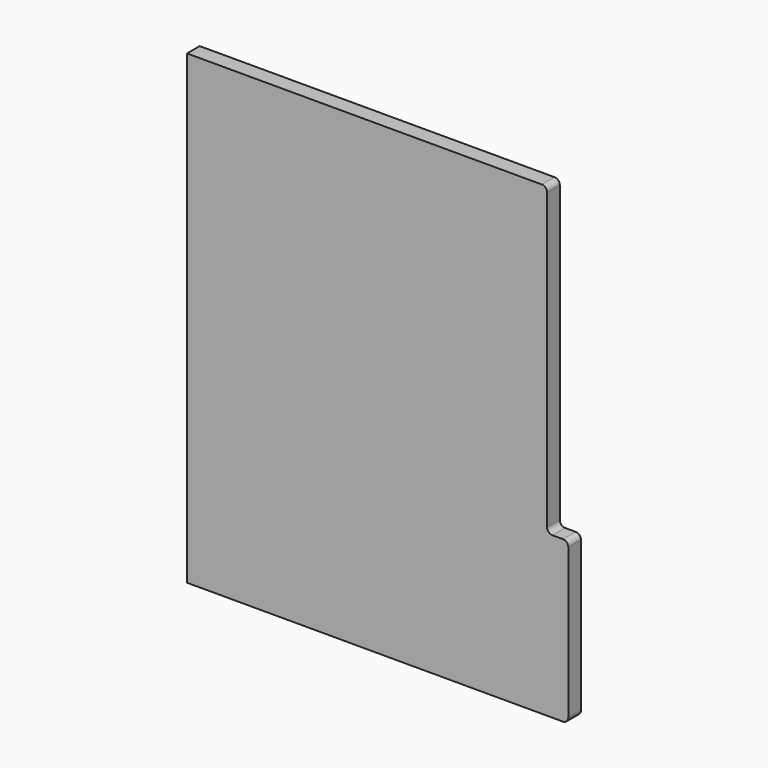
from build123d import *

# Parameters (mm, degrees)
F0_W     = 215.9
F0_H     = 279.4
F1_DEPTH = 9.525
F2_W     = 12.7
F2_H     = 96.3083333333
F3_DEPTH = 9.525
F4_R     = 3.175


with BuildPart() as f1:
    # F0 (on Front) → F1 (new body)
    with BuildSketch(Plane.XZ):
        Rectangle(F0_W, F0_H)
    extrude(amount=F1_DEPTH)

    # F2 (on Front) → F3 (join, through all)
    with BuildSketch(Plane.XZ):
        with Locations((114.3, -91.5458333333)):
            Rectangle(F2_W, F2_H)
    extrude(amount=F3_DEPTH)

    # F4
    f4_edges = [f1.edges().sort_by_distance(p)[0] for p in [
        (107.95, -4.7625, 139.7),
        (107.95, -4.7625, -43.391667),
        (120.65, -4.7625, -43.391667),
        (120.65, -4.7625, -139.7),
    ]]
    fillet(f4_edges, radius=F4_R)


solid = f1.part
